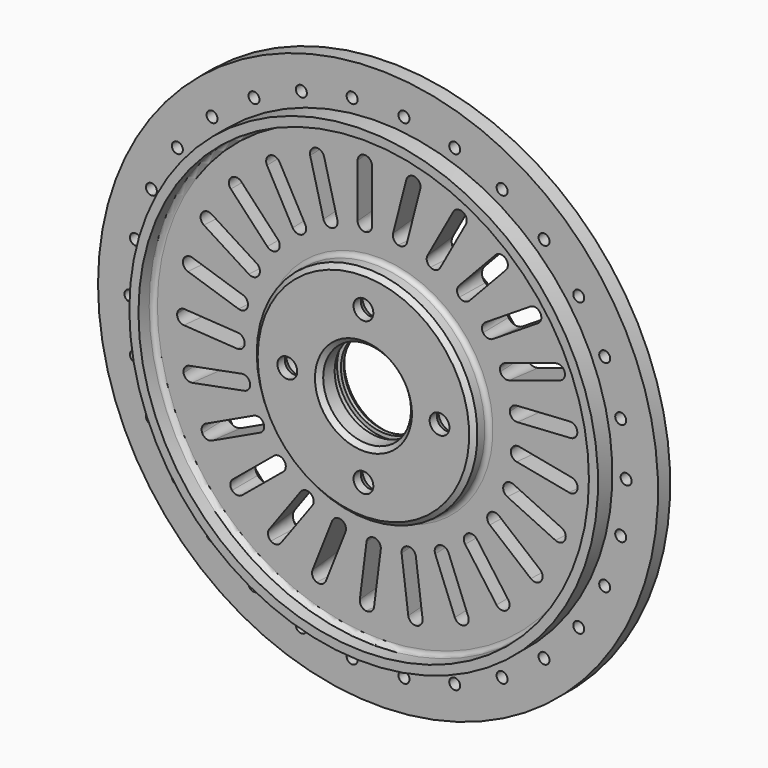
from build123d import *

# Parameters (mm, degrees)
F3_R             = 3.6
F4_DEPTH         = 50
F4_COPIES_COUNT  = 30
F6_COPIES_COUNT  = 4
F7_SIZE          = 3
F8_R             = 135
F8_R_2           = 85
F9_DEPTH         = 3
F11_DEPTH        = 50
F11_TAPER        = 5
F11_COPIES_COUNT = 25


# Not quite as in the source:
# - a pattern or mirror of a feature is missing from the dataset's text; its kind, count and spacing are read off the source's solid


with BuildPart() as f1:
    # F0 (on Top) → F1 (revolve)
    with BuildSketch(Plane.XY):
        with BuildLine():
            ThreePointArc((-75.5, 12), (-73.3786796564, 11.1213203436), (-72.5, 9))
            Line((-72.5, 9), (-72.5, 0))
            Line((-72.5, 0), (-28.85, 0))
            Line((-28.85, 0), (-28.85, 12.4))
            Line((-28.85, 12.4), (-31.45, 12.4))
            Line((-31.45, 12.4), (-31.45, 17.6))
            Line((-31.45, 17.6), (-28.85, 17.6))
            Line((-28.85, 17.6), (-28.85, 20))
            Line((-28.85, 20), (-30, 20))
            ThreePointArc((-30, 20), (-30.7071067812, 20.2928932188), (-31, 21))
            Line((-31, 21), (-31, 23))
            Line((-31, 23), (-67.5, 37))
            Line((-67.5, 37), (-154, 37))
            Line((-154, 37), (-154, 22))
            Line((-154, 22), (-184, 22))
            Line((-184, 22), (-184, 12))
            Line((-184, 12), (-154, 12))
            Line((-154, 12), (-154, 0.2))
            Line((-154, 0.2), (-148, 0.2))
            Line((-148, 0.2), (-148, 9))
            ThreePointArc((-148, 9), (-147.1213203436, 11.1213203436), (-145, 12))
            Line((-145, 12), (-75.5, 12))
        make_face()
    revolve(axis=Axis((0, 8.013517431, 0), (0, -1, 0)))

    # F3 (on Front) → F4 (cut)
    with BuildSketch(Plane.XZ):
        with Locations((163, 0)):
            Circle(F3_R)
    f4 = extrude(amount=-F4_DEPTH, mode=Mode.SUBTRACT)

    # F4_copies: F4 ×30 about axis
    f4_copies_axis = Axis((0, 0, 0), (0, 1, 0))
    for i in range(1, F4_COPIES_COUNT):
        add(f4.rotate(f4_copies_axis, i * 360 / F4_COPIES_COUNT), mode=Mode.SUBTRACT)

    # F5 (on Right) → F6 (revolve, cut)
    with BuildSketch(Plane.YZ):
        Polygon((0, 56.5), (0, 50), (51.0571013514, 50), (51.0571013514, 59), (10.3301270189, 59), (6, 56.5), align=None)
    f6 = revolve(axis=Axis((0, 25.5285506757, 50), (0, 1, 0)), mode=Mode.SUBTRACT)

    # F6_copies: F6 ×4 about axis
    f6_copies_axis = Axis((0, 0, 0), (0, 1, 0))
    for i in range(1, F6_COPIES_COUNT):
        add(f6.rotate(f6_copies_axis, i * 360 / F6_COPIES_COUNT), mode=Mode.SUBTRACT)

    # F7
    f7_edges = [f1.edges().sort_by_distance(p)[0] for p in [
        (72.5, 0, 0),
        (28.85, 0, 0),
    ]]
    chamfer(f7_edges, length=F7_SIZE)

    # F8 (on offset) → F9 (cut, through all)
    with BuildSketch(Plane.XZ.offset(-38)):
        Circle(F8_R)
        Circle(F8_R_2, mode=Mode.SUBTRACT)
    extrude(amount=F9_DEPTH, mode=Mode.SUBTRACT)

    # F10 (on offset) → F11 (cut)
    with BuildSketch(Plane.XZ.offset(-38)):
        with BuildLine():
            ThreePointArc((-8.7, 134), (-13.6497474683, 131.9497474683), (-15.7, 127))
            Line((-15.7, 127), (-15.7, 92))
            ThreePointArc((-15.7, 92), (-13.6497474683, 87.0502525317), (-8.7, 85))
            ThreePointArc((-8.7, 85), (-3.7502525317, 87.0502525317), (-1.7, 92))
            Line((-1.7, 92), (-1.7, 127))
            ThreePointArc((-1.7, 127), (-3.7502525317, 131.9497474683), (-8.7, 134))
        make_face()
    f11 = extrude(amount=F11_DEPTH, taper=F11_TAPER, mode=Mode.SUBTRACT)

    # F11_copies: F11 ×25 about axis
    f11_copies_axis = Axis((0, 0, 0), (0, 1, 0))
    for i in range(1, F11_COPIES_COUNT):
        add(f11.rotate(f11_copies_axis, i * 360 / F11_COPIES_COUNT), mode=Mode.SUBTRACT)


solid = f1.part
